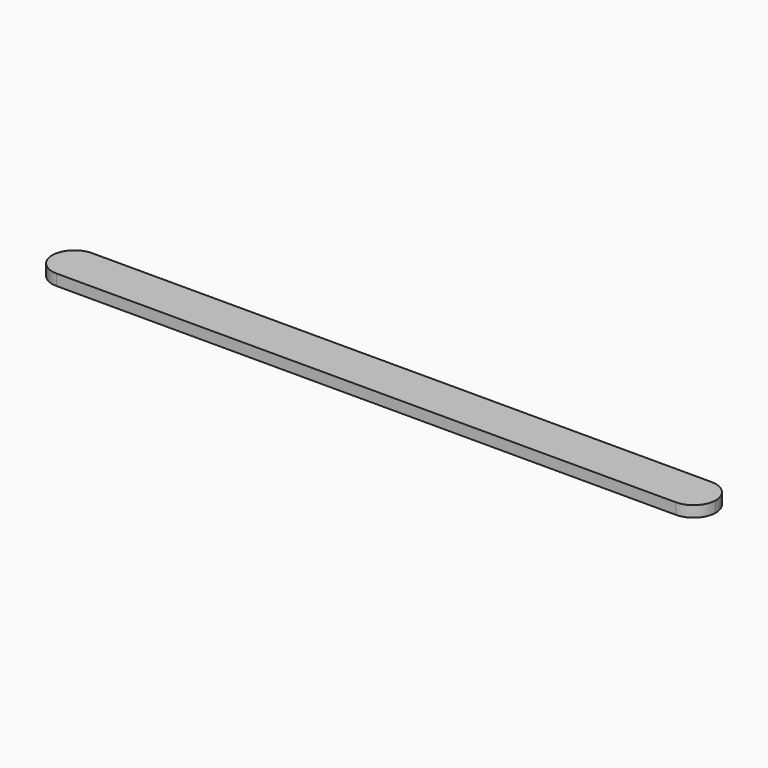
from build123d import *

# Parameters (mm, degrees)
F1_DEPTH = 3.175
F2_W     = 9.525
F2_H     = 3.175
F3_DEPTH = 152.4
F5_DEPTH = 9.525


# Not quite as in the source:
# - a length typed as a fraction of an inch, garbled in the dataset ("3 / 203.2 mm" for 3/8 in), is restored
# - a feature names something its author has since deleted; it is built from what else it names


with BuildPart() as f1:
    # F0 (on Top) → F1 (new body, symmetric)
    with BuildSketch(Plane.XY):
        with BuildLine():
            Line((-152.4, 12.7), (-177.8, 12.7))
            ThreePointArc((-177.8, 12.7), (-186.780256, 8.980256), (-190.5, 0))
            ThreePointArc((-190.5, 0), (-186.780256, -8.980256), (-177.8, -12.7))
            Line((-177.8, -12.7), (-152.4, -12.7))
            Line((-152.4, -12.7), (152.4, -12.7))
            Line((152.4, -12.7), (177.8, -12.7))
            ThreePointArc((177.8, -12.7), (186.780256, -8.980256), (190.5, 0))
            ThreePointArc((190.5, 0), (186.780256, 8.980256), (177.8, 12.7))
            Line((177.8, 12.7), (152.4, 12.7))
            Line((152.4, 12.7), (-152.4, 12.7))
        make_face()
    extrude(amount=F1_DEPTH, both=True)

    # F2 (on Right) → F3 (cut, symmetric)
    with BuildSketch(Plane.YZ):
        with Locations((0, -1.5875)):
            Rectangle(F2_W, F2_H)
    extrude(amount=F3_DEPTH, both=True, mode=Mode.SUBTRACT)

    # F4 (on face) → F5 (cut)
    with BuildSketch(Plane(origin=(0, -4.7625, 0), x_dir=(-1, 0, 0), z_dir=(0, 1, 0))):
        Polygon((161.925, -3.175), (152.4, 0), (152.4, -3.175), align=None)
        Polygon((-152.4, -3.175), (-152.4, 0), (-161.925, -3.175), align=None)
    extrude(amount=F5_DEPTH, mode=Mode.SUBTRACT)


solid = f1.part
